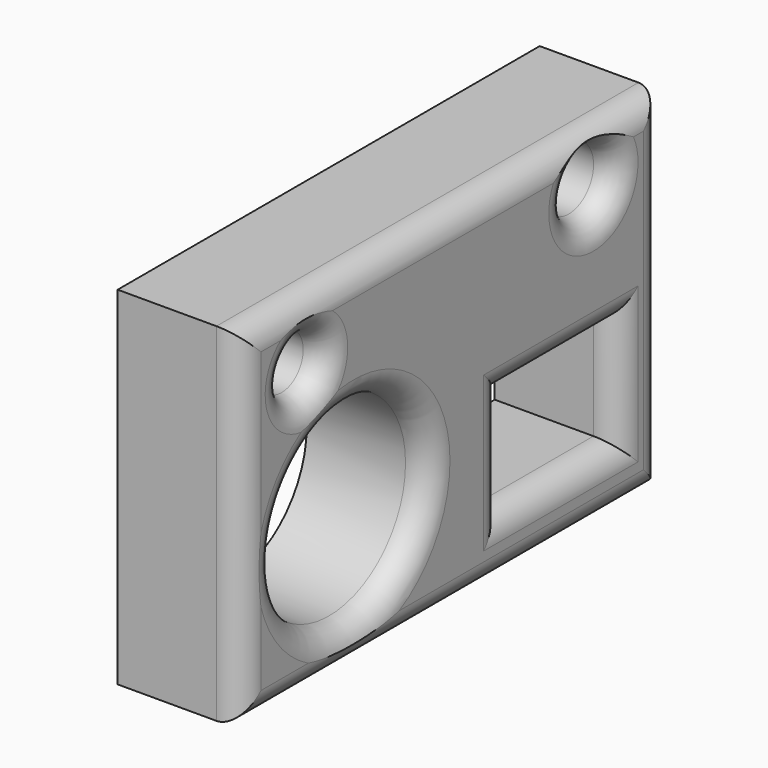
from build123d import *

# Parameters (mm, degrees)
F0_W         = 108.5126549006
F0_H         = 71.473672986
F0_R         = 19.6812167499
F0_W_2       = 29.5154461637
F0_H_2       = 21.7025321908
F0_R_2       = 5.5283506547
F0_R_3       = 6.3923279955
F1_DEPTH     = 25.4
F2_T1_DEPTH  = 29.5154461637
F2_T3_DEPTH  = 133.9126549006
F2_T5_DEPTH  = 96.873672986
F2_T7_DEPTH  = 21.7025321908
F2_T19_DEPTH = 34.4025321908
F2_T23_DEPTH = 42.2154461637
F2_T30_DEPTH = 42.2154461637
F2_T34_DEPTH = 34.4025321908
F2_T41_DEPTH = 34.4025321908
F2_T45_DEPTH = 42.2154461637
F2_T52_DEPTH = 34.4025321908
F2_T56_DEPTH = 42.2154461637


# Not quite as in the source:
# - a fillet or chamfer that OpenCascade refuses, or shapes differently, is made with other operations: its cross-section is extruded or revolved along the edge and cut away or added


with BuildPart() as f1:
    # F0 (on Right) → F1 (new body)
    with BuildSketch(Plane.YZ):
        with Locations((-1.3021528721, -0.2893656492)):
            Rectangle(F0_W, F0_H)
        with Locations((-26.6217719764, -9.1150635853)):
            Circle(F0_R, mode=Mode.SUBTRACT)
        with Locations((26.6217733733, -13.0215191748)):
            Rectangle(F0_W_2, F0_H_2, mode=Mode.SUBTRACT)
        with Locations((-38.775190711, 22.1365820616)):
            Circle(F0_R_2, mode=Mode.SUBTRACT)
        with Locations((35.01342237, 25.3196209669)):
            Circle(F0_R_3, mode=Mode.SUBTRACT)
    extrude(amount=F1_DEPTH)

    # F2: fillet of radius 5.08 on 11 edges, made by hand

    # F2_s2 → F2_t1 (cut)
    with BuildSketch(Plane.XZ.offset(-41.3794964552)):
        with BuildLine():
            ThreePointArc((20.32, -2.1702530794), (23.9121024484, -0.6823555278), (25.4, 2.9097469206))
            Line((25.4, 2.9097469206), (25.4, -2.1702530794))
            Line((25.4, -2.1702530794), (20.32, -2.1702530794))
        make_face()
        with BuildLine():
            ThreePointArc((20.32, -23.8727852702), (23.9121024484, -25.3606828218), (25.4, -28.9527852702))
            Line((25.4, -28.9527852702), (25.4, -23.8727852702))
            Line((25.4, -23.8727852702), (20.32, -23.8727852702))
        make_face()
    extrude(amount=F2_T1_DEPTH, mode=Mode.SUBTRACT)

    # F2_s4 → F2_t3 (cut)
    with BuildSketch(Plane.XZ.offset(-65.6541745782)):
        with BuildLine():
            ThreePointArc((20.32, 35.4474708438), (23.9121024484, 33.9595732922), (25.4, 30.3674708438))
            Line((25.4, 30.3674708438), (25.4, 35.4474708438))
            Line((25.4, 35.4474708438), (20.32, 35.4474708438))
        make_face()
        with BuildLine():
            ThreePointArc((20.32, -36.0262021422), (23.9121024484, -34.5383045907), (25.4, -30.9462021422))
            Line((25.4, -30.9462021422), (25.4, -36.0262021422))
            Line((25.4, -36.0262021422), (20.32, -36.0262021422))
        make_face()
    extrude(amount=F2_T3_DEPTH, mode=Mode.SUBTRACT)

    # F2_s6 → F2_t5 (cut)
    with BuildSketch(Plane.XY.offset(-48.7262021422)):
        with BuildLine():
            ThreePointArc((20.32, -55.5584803224), (23.9121024484, -54.0705827708), (25.4, -50.4784803224))
            Line((25.4, -50.4784803224), (25.4, -55.5584803224))
            Line((25.4, -55.5584803224), (20.32, -55.5584803224))
        make_face()
        with BuildLine():
            ThreePointArc((20.32, 52.9541745782), (23.9121024484, 51.4662770266), (25.4, 47.8741745782))
            Line((25.4, 47.8741745782), (25.4, 52.9541745782))
            Line((25.4, 52.9541745782), (20.32, 52.9541745782))
        make_face()
    extrude(amount=F2_T5_DEPTH, mode=Mode.SUBTRACT)

    # F2_s8 → F2_t7 (cut)
    with BuildSketch(Plane.XY.offset(-23.8727852702)):
        with BuildLine():
            ThreePointArc((20.32, 11.8640502915), (23.9121024484, 10.3761527399), (25.4, 6.7840502915))
            Line((25.4, 6.7840502915), (25.4, 11.8640502915))
            Line((25.4, 11.8640502915), (20.32, 11.8640502915))
        make_face()
        with BuildLine():
            ThreePointArc((20.32, 41.3794964552), (23.9121024484, 42.8673940068), (25.4, 46.4594964552))
            Line((25.4, 46.4594964552), (25.4, 41.3794964552))
            Line((25.4, 41.3794964552), (20.32, 41.3794964552))
        make_face()
    extrude(amount=F2_T7_DEPTH, mode=Mode.SUBTRACT)

    # F2_s9 → F2_t10 (revolve, cut)
    with BuildSketch(Plane.XY.offset(-9.1150635853)):
        with BuildLine():
            ThreePointArc((20.32, -6.9405552264), (23.9121024484, -5.4526576749), (25.4, -1.8605552264))
            Line((25.4, -1.8605552264), (25.4, -6.9405552264))
            Line((25.4, -6.9405552264), (20.32, -6.9405552264))
        make_face()
    revolve(axis=Axis((25.4, -26.6217719764, -9.1150635853), (1, 0, 0)), mode=Mode.SUBTRACT)

    # F2_s11 → F2_t12 (revolve, cut)
    with BuildSketch(Plane.XY.offset(22.1365820616)):
        with BuildLine():
            ThreePointArc((20.32, -33.2468400563), (23.9121024484, -31.7589425047), (25.4, -28.1668400563))
            Line((25.4, -28.1668400563), (25.4, -33.2468400563))
            Line((25.4, -33.2468400563), (20.32, -33.2468400563))
        make_face()
    revolve(axis=Axis((25.4, -38.775190711, 22.1365820616), (1, 0, 0)), mode=Mode.SUBTRACT)

    # F2_s13 → F2_t14 (revolve, cut)
    with BuildSketch(Plane.XY.offset(25.3196209669)):
        with BuildLine():
            ThreePointArc((20.32, 41.4057503654), (23.9121024484, 42.893647917), (25.4, 46.4857503654))
            Line((25.4, 46.4857503654), (25.4, 41.4057503654))
            Line((25.4, 41.4057503654), (20.32, 41.4057503654))
        make_face()
    revolve(axis=Axis((25.4, 35.01342237, 25.3196209669), (1, 0, 0)), mode=Mode.SUBTRACT)


with BuildPart() as f2_tool17:
    # F2_s18 → F2_t19 (new body)
    with BuildSketch(Plane.XY.offset(-23.8727852702)):
        with BuildLine():
            ThreePointArc((20.32, 11.8640502915), (23.9121024484, 10.3761527399), (25.4, 6.7840502915))
            Line((25.4, 6.7840502915), (25.4, 11.8640502915))
            Line((25.4, 11.8640502915), (20.32, 11.8640502915))
        make_face()
    extrude(amount=F2_T19_DEPTH)

    split(bisect_by=Plane.XY.offset(-2.1702530794), keep=Keep.TOP)


with BuildPart() as f2_tool21:
    # F2_s22 → F2_t23 (new body)
    with BuildSketch(Plane.XZ.offset(0.8359497085)):
        with BuildLine():
            ThreePointArc((20.32, -2.1702530794), (23.9121024484, -0.6823555278), (25.4, 2.9097469206))
            Line((25.4, 2.9097469206), (25.4, -2.1702530794))
            Line((25.4, -2.1702530794), (20.32, -2.1702530794))
        make_face()
    extrude(amount=-F2_T23_DEPTH)

    split(bisect_by=Plane.XZ.offset(-11.8640502915), keep=Keep.TOP)


with BuildPart() as f2_tool17_1:
    add(f2_tool17.part)

    # F2_t25: intersect F2_tool21
    add(f2_tool21.part, mode=Mode.INTERSECT)


with BuildPart() as f1_1:
    add(f1.part)

    # F2_t15: cut F2_tool17
    add(f2_tool17_1.part, mode=Mode.SUBTRACT)


with BuildPart() as f2_tool28:
    # F2_s29 → F2_t30 (new body)
    with BuildSketch(Plane.XZ.offset(-11.8640502915)):
        with BuildLine():
            ThreePointArc((20.32, -2.1702530794), (23.9121024484, -0.6823555278), (25.4, 2.9097469206))
            Line((25.4, 2.9097469206), (25.4, -2.1702530794))
            Line((25.4, -2.1702530794), (20.32, -2.1702530794))
        make_face()
    extrude(amount=-F2_T30_DEPTH)

    split(bisect_by=Plane.XZ.offset(-41.3794964552), keep=Keep.BOTTOM)


with BuildPart() as f2_tool32:
    # F2_s33 → F2_t34 (new body)
    with BuildSketch(Plane.XY.offset(10.5297469206)):
        with BuildLine():
            ThreePointArc((20.32, 41.3794964552), (23.9121024484, 42.8673940068), (25.4, 46.4594964552))
            Line((25.4, 46.4594964552), (25.4, 41.3794964552))
            Line((25.4, 41.3794964552), (20.32, 41.3794964552))
        make_face()
    extrude(amount=-F2_T34_DEPTH)

    split(bisect_by=Plane.XY.offset(-2.1702530794), keep=Keep.TOP)


with BuildPart() as f2_tool28_1:
    add(f2_tool28.part)

    # F2_t36: intersect F2_tool32
    add(f2_tool32.part, mode=Mode.INTERSECT)


with BuildPart() as f1_2:
    add(f1_1.part)

    # F2_t26: cut F2_tool28
    add(f2_tool28_1.part, mode=Mode.SUBTRACT)


with BuildPart() as f2_tool39:
    # F2_s40 → F2_t41 (new body)
    with BuildSketch(Plane.XY.offset(-36.5727852702)):
        with BuildLine():
            ThreePointArc((20.32, 11.8640502915), (23.9121024484, 10.3761527399), (25.4, 6.7840502915))
            Line((25.4, 6.7840502915), (25.4, 11.8640502915))
            Line((25.4, 11.8640502915), (20.32, 11.8640502915))
        make_face()
    extrude(amount=F2_T41_DEPTH)

    split(bisect_by=Plane.XY.offset(-23.8727852702), keep=Keep.BOTTOM)


with BuildPart() as f2_tool43:
    # F2_s44 → F2_t45 (new body)
    with BuildSketch(Plane.XZ.offset(-41.3794964552)):
        with BuildLine():
            ThreePointArc((20.32, -23.8727852702), (23.9121024484, -25.3606828218), (25.4, -28.9527852702))
            Line((25.4, -28.9527852702), (25.4, -23.8727852702))
            Line((25.4, -23.8727852702), (20.32, -23.8727852702))
        make_face()
    extrude(amount=F2_T45_DEPTH)

    split(bisect_by=Plane.XZ.offset(-11.8640502915), keep=Keep.TOP)


with BuildPart() as f2_tool39_1:
    add(f2_tool39.part)

    # F2_t47: intersect F2_tool43
    add(f2_tool43.part, mode=Mode.INTERSECT)


with BuildPart() as f1_3:
    add(f1_2.part)

    # F2_t37: cut F2_tool39
    add(f2_tool39_1.part, mode=Mode.SUBTRACT)


with BuildPart() as f2_tool50:
    # F2_s51 → F2_t52 (new body)
    with BuildSketch(Plane.XY.offset(-2.1702530794)):
        with BuildLine():
            ThreePointArc((20.32, 41.3794964552), (23.9121024484, 42.8673940068), (25.4, 46.4594964552))
            Line((25.4, 46.4594964552), (25.4, 41.3794964552))
            Line((25.4, 41.3794964552), (20.32, 41.3794964552))
        make_face()
    extrude(amount=-F2_T52_DEPTH)

    split(bisect_by=Plane.XY.offset(-23.8727852702), keep=Keep.BOTTOM)


with BuildPart() as f2_tool54:
    # F2_s55 → F2_t56 (new body)
    with BuildSketch(Plane.XZ.offset(-54.0794964552)):
        with BuildLine():
            ThreePointArc((20.32, -23.8727852702), (23.9121024484, -25.3606828218), (25.4, -28.9527852702))
            Line((25.4, -28.9527852702), (25.4, -23.8727852702))
            Line((25.4, -23.8727852702), (20.32, -23.8727852702))
        make_face()
    extrude(amount=F2_T56_DEPTH)

    split(bisect_by=Plane.XZ.offset(-41.3794964552), keep=Keep.BOTTOM)


with BuildPart() as f2_tool50_1:
    add(f2_tool50.part)

    # F2_t58: intersect F2_tool54
    add(f2_tool54.part, mode=Mode.INTERSECT)


with BuildPart() as f1_4:
    add(f1_3.part)

    # F2_t48: cut F2_tool50
    add(f2_tool50_1.part, mode=Mode.SUBTRACT)


solid = f1_4.part
